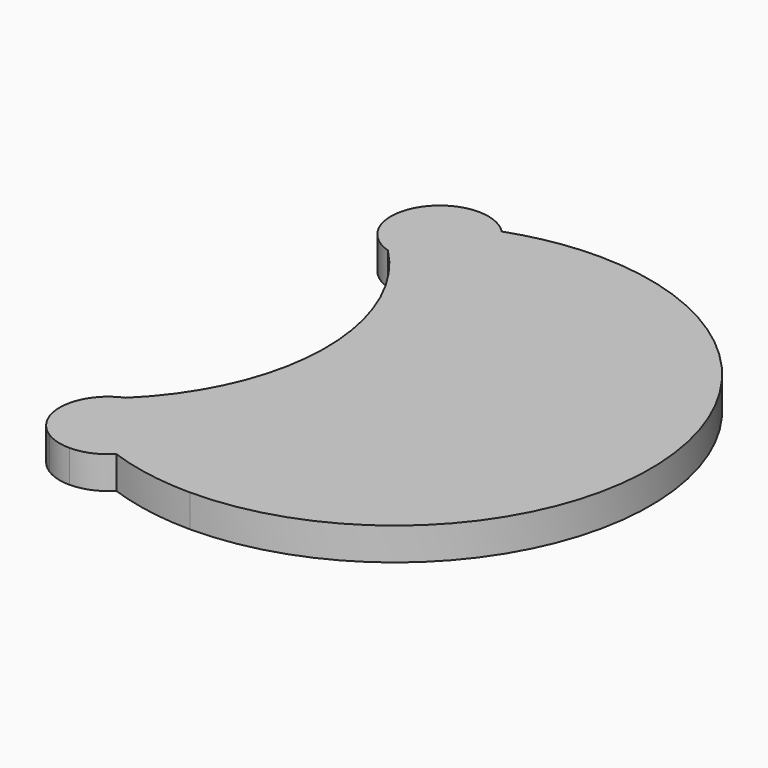
from build123d import *

# Parameters (mm, degrees)
F1_DEPTH = 6.35


# Not quite as in the source:
# - a feature names something its author has since deleted; it is built from what else it names


with BuildPart() as f1:
    # F0 (on Top) → F1 (new body)
    with BuildSketch(Plane.XY):
        with BuildLine():
            ThreePointArc((-20.6136406437, -48.4949748961), (-18.1522527003, -49.6160033902), (-15.474999986, -50))
            ThreePointArc((-15.474999986, -50), (-11.7658348983, -49.248124828), (-8.64225073, -47.1112009021))
            ThreePointArc((-8.64225073, -47.1112009021), (-0.3913128261, -49.2725077899), (8.1069210399, -50))
            ThreePointArc((8.1069210399, -50), (58.1069208781, 4.4e-08), (8.1069209519, 50))
            ThreePointArc((8.1069209519, 50), (-0.3913128695, 49.2725077824), (-8.64225073, 47.1112009021))
            ThreePointArc((-8.64225073, 47.1112009021), (-11.7658349048, 49.2481248308), (-15.475, 50))
            ThreePointArc((-15.475, 50), (-17.9163659919, 49.6818103648), (-20.1946207283, 48.7485001771))
            ThreePointArc((-20.1946207283, 48.7485001771), (-23.7115044996, 45.2588915778), (-25, 40.4749999628))
            ThreePointArc((-25, 40.4749999628), (-24.7547421233, 38.3274406584), (-24.0315987301, 36.2904757532))
            ThreePointArc((-24.0315987301, 36.2904757532), (-21.6846733781, 33.2524255603), (-18.3290256128, 31.3876371921))
            ThreePointArc((-18.3290256128, 31.3876371921), (-5.6085763504, -0.3160997755), (-19.1387594108, -31.6828164271))
            ThreePointArc((-19.1387594108, -31.6828164271), (-21.6396911965, -33.2139940469), (-23.5563206429, -35.433385014))
            ThreePointArc((-23.5563206429, -35.433385014), (-24.6319701355, -37.8528781611), (-25, -40.475))
            ThreePointArc((-25, -40.475), (-23.8317690267, -45.0455619386), (-20.6136406437, -48.4949748961))
        make_face()
    extrude(amount=F1_DEPTH)


solid = f1.part
